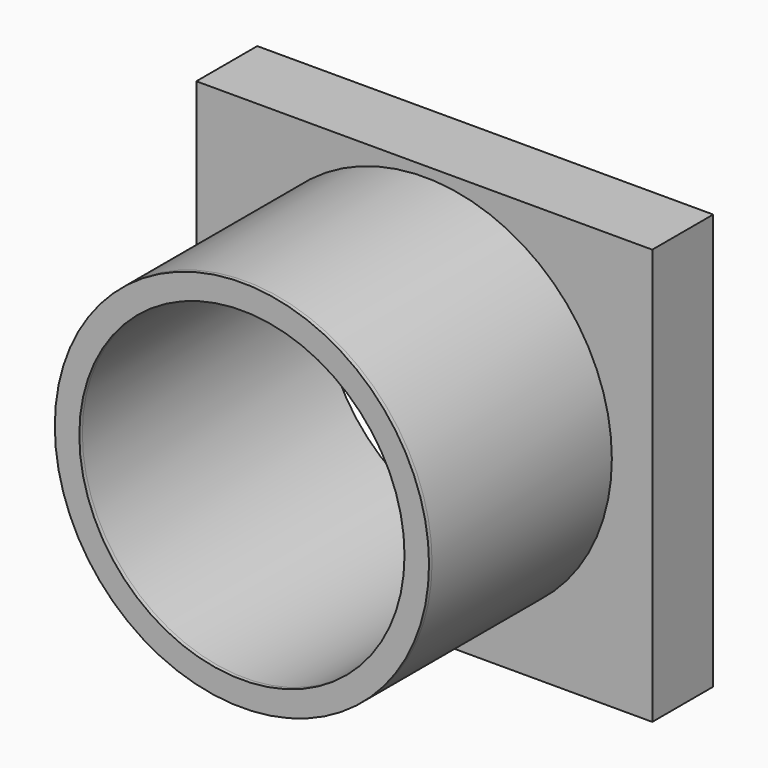
from build123d import *

# Parameters (mm, degrees)
F0_R        = 62.3961855018
F0_R_2      = 54.2236772846
F1_DEPTH    = 25.4
F2_DEPTH    = 50.8
F0_W        = 152.0332619548
F0_H        = 138.626947999
F2_FACE_R   = 62.3961855018
F2_FACE_R_2 = 54.2236772846
F3_DEPTH    = 25.4
F4_DEPTH    = 1.27


with BuildPart() as f1:
    # F0 (on Front) → F1 (new body)
    with BuildSketch(Plane.XZ):
        Circle(F0_R)
        Circle(F0_R_2, mode=Mode.SUBTRACT)
    extrude(amount=F1_DEPTH)

    # F2 (add): faces of the model
    f2_faces = [f1.faces().sort_by_distance(p)[0] for p in [
        (-60.6313548663, -25.4, 0),
        (-60.6313548663, 0, 0),
    ]]
    extrude(f2_faces, amount=F2_DEPTH, dir=(0, -1, 0))

    # F0 (on Front) + F2_face (on face) → F3 (join)
    with BuildSketch(Plane.XZ):
        with Locations((-0.1426227391, -3.565505147)):
            Rectangle(F0_W, F0_H)
        Circle(F0_R, mode=Mode.SUBTRACT)
    with BuildSketch(Plane.XZ.offset(76.2)):
        Circle(F2_FACE_R)
        Circle(F2_FACE_R_2, mode=Mode.SUBTRACT)
    extrude(amount=F3_DEPTH)


with BuildPart() as f4:
    # F4 (new): a face of the model
    f4_faces = [f1.part.faces().sort_by_distance(p)[0] for p in [
        (-60.6313548663, -101.6, 0),
    ]]
    extrude(f4_faces, amount=-F4_DEPTH)


solid = Compound([f1.part, f4.part])
